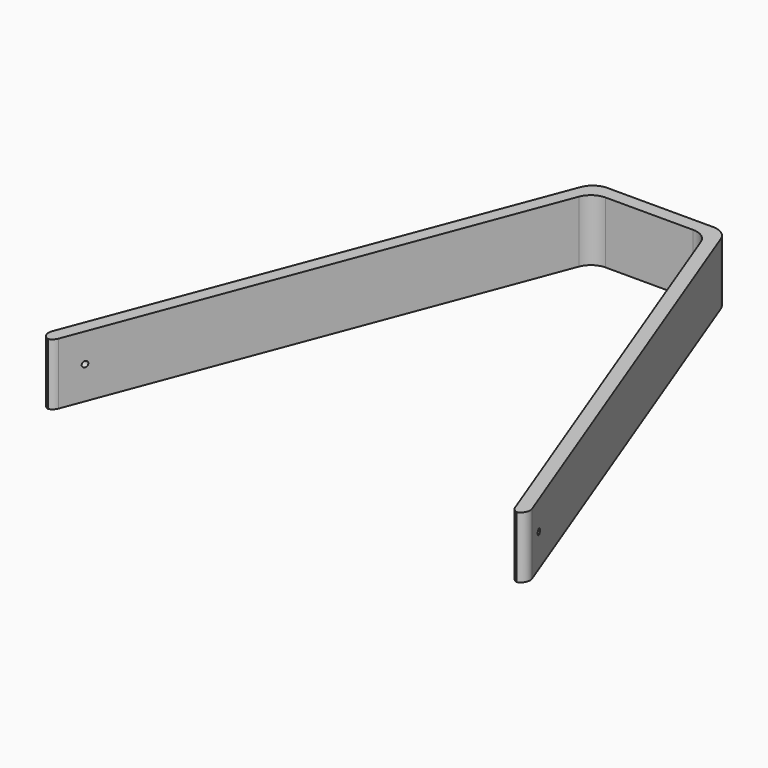
from build123d import *

# Parameters (mm, degrees)
F1_DEPTH      = 12.7
F2_T1_DEPTH   = 19.2753145827
F2_T3_DEPTH   = 26.4979139795
F3_R          = 3.81
F4_R          = 0.5908054237
F5_DEPTH      = 57.15
F5_DEPTH_BACK = 73.914


# Not quite as in the source:
# - a fillet or chamfer that OpenCascade refuses, or shapes differently, is made with other operations: its cross-section is extruded or revolved along the edge and cut away or added


with BuildPart() as f1:
    # F0 (on Top) → F1 (new body)
    with BuildSketch(Plane.XY):
        Polygon((13.5222204362, 66.8438002467), (0, 66.8438002467), (-13.5222204362, 66.8438002467), (-50.4813892832, -30.6380242109), (-47.5520528853, -30.6380242109), (-11.6511627941, 64.052532285), (0, 64.052532285), (11.6511627941, 64.052532285), (47.5520528853, -30.6380242109), (50.4813892832, -30.6380242109), align=None)
    extrude(amount=F1_DEPTH)

    # F2: fillet of radius 1.905 on 4 edges, made by hand

    # F2_s2 → F2_t1 (cut)
    with BuildSketch(Plane.XY.offset(-3.2876572913)):
        with BuildLine():
            ThreePointArc((-47.0858443706, -29.4083738154), (-47.784876456, -30.3007560114), (-48.8671158018, -30.6380242109))
            Line((-48.8671158018, -30.6380242109), (-47.5520528853, -30.6380242109))
            Line((-47.5520528853, -30.6380242109), (-47.0858443706, -29.4083738154))
        make_face()
        with BuildLine():
            ThreePointArc((47.0858443706, -29.4083738154), (47.784876456, -30.3007560114), (48.8671158018, -30.6380242109))
            Line((48.8671158018, -30.6380242109), (47.5520528853, -30.6380242109))
            Line((47.5520528853, -30.6380242109), (47.0858443706, -29.4083738154))
        make_face()
    extrude(amount=F2_T1_DEPTH, mode=Mode.SUBTRACT)

    # F2_s4 → F2_t3 (cut)
    with BuildSketch(Plane.XY.offset(-6.8989569898)):
        with BuildLine():
            ThreePointArc((-47.7218064873, -30.6380242109), (-49.2895382878, -29.8152635568), (-49.5030779186, -28.0576746065))
            Line((-49.5030779186, -28.0576746065), (-50.4813892832, -30.6380242109))
            Line((-50.4813892832, -30.6380242109), (-47.7218064873, -30.6380242109))
        make_face()
        with BuildLine():
            ThreePointArc((49.5030779186, -28.0576746065), (49.2895382878, -29.8152635568), (47.7218064873, -30.6380242109))
            Line((47.7218064873, -30.6380242109), (50.4813892832, -30.6380242109))
            Line((50.4813892832, -30.6380242109), (49.5030779186, -28.0576746065))
        make_face()
    extrude(amount=F2_T3_DEPTH, mode=Mode.SUBTRACT)

    # F3
    f3_edges = [f1.edges().sort_by_distance(p)[0] for p in [
        (13.52222, 66.8438, 6.35),
        (-13.52222, 66.8438, 6.35),
        (-11.651163, 64.052532, 6.35),
        (11.651163, 64.052532, 6.35),
    ]]
    fillet(f3_edges, radius=F3_R)

    # F4 (on Right) → F5 (cut, two sides)
    with BuildSketch(Plane.YZ) as f5_sk:
        with Locations((-24.7479453683, 6.7547173239)):
            Circle(F4_R)
    extrude(amount=-F5_DEPTH, mode=Mode.SUBTRACT)
    extrude(f5_sk.sketch, amount=F5_DEPTH_BACK, mode=Mode.SUBTRACT)


solid = f1.part
